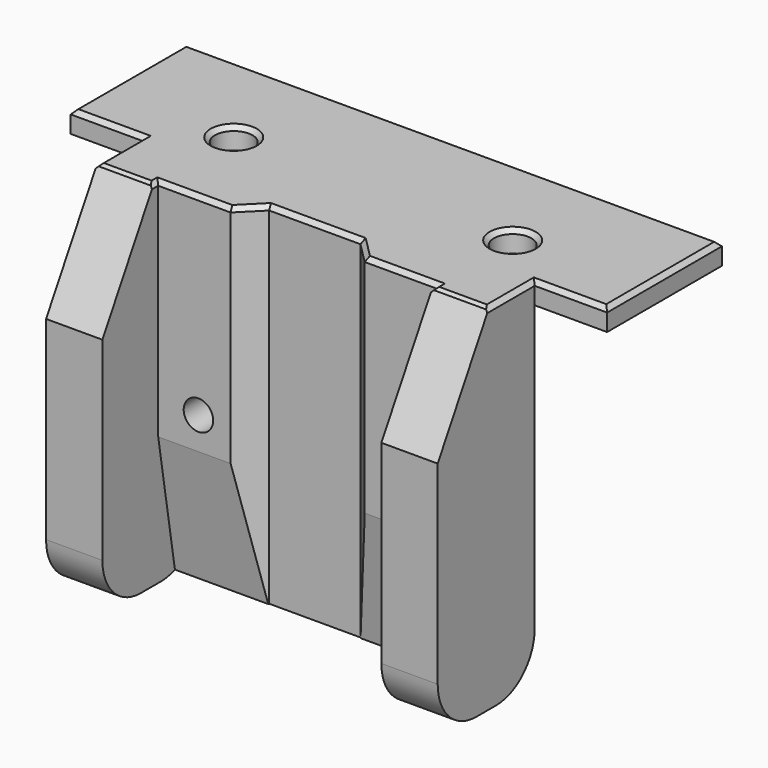
from build123d import *

# Parameters (mm, degrees)
F0_W           = 13.375
F0_H           = 2
F1_DEPTH       = 25
F2_R           = 1.75
F3_DEPTH       = 2
F4_W           = 11.3
F4_H           = 33
F5_DEPTH       = 18.25
F6_W           = 26
F6_H           = 6.5
F7_DEPTH       = 33
F9_DEPTH       = 33
F11_DEPTH      = 13
F11_DEPTH_BACK = 13
F12_R          = 1.375
F13_DEPTH      = 4.8
F14_W          = 5.5
F14_H          = 5.5
F15_DEPTH      = 1.5
F16_T1_DEPTH   = 27.75
F16_T3_DEPTH   = 27.75
F16_T5_DEPTH   = 59
F17_T1_DEPTH   = 59.021567647
F17_T3_DEPTH   = 59.021567647
F18_T1_DEPTH   = 15.4323463904
F18_T3_DEPTH   = 52.0573463904
F18_T5_DEPTH   = 7.7786731952
F18_T7_DEPTH   = 6.3286731952
F18_T9_DEPTH   = 6.4746360003
F18_T11_DEPTH  = 1.5286731952
F18_T13_DEPTH  = 7.7786731952
F18_T15_DEPTH  = 7.7786731952
F18_T17_DEPTH  = 6.4746360003
F18_T19_DEPTH  = 7.7786731952
F18_T24_DEPTH  = 4.8857735151
F18_T29_DEPTH  = 10.5573463904
F18_T35_DEPTH  = 4.8857735151
F18_T45_DEPTH  = 7.7786731952
F18_T49_DEPTH  = 7.3573463904
F18_T56_DEPTH  = 2.5573463904
F18_T60_DEPTH  = 8.8073463904
F18_T67_DEPTH  = 10.5573463904
F18_T71_DEPTH  = 4.8857735151
F18_T78_DEPTH  = 4.8857735151
F18_T82_DEPTH  = 10.5573463904
F18_T89_DEPTH  = 2.5573463904
F18_T93_DEPTH  = 8.8073463904
F18_T100_DEPTH = 7.7786731952
F18_T104_DEPTH = 7.3573463904


# Not quite as in the source:
# - a fillet or chamfer that OpenCascade refuses, or shapes differently, is made with other operations: its cross-section is extruded or revolved along the edge and cut away or added


with BuildPart() as f1:
    # F0 (on Right) → F1 (new body, symmetric)
    with BuildSketch(Plane.YZ):
        with Locations((6.6875, 1)):
            Rectangle(F0_W, F0_H)
    extrude(amount=F1_DEPTH, both=True)

    # F2 (on face) → F3 (cut, through all)
    with BuildSketch(Plane.XY.offset(2)):
        with Locations((-13, 4)):
            Circle(F2_R)
        with Locations((13, 4)):
            Circle(F2_R)
    extrude(amount=-F3_DEPTH, mode=Mode.SUBTRACT)

    # F4 (on Right) → F5 (join, symmetric)
    with BuildSketch(Plane.YZ):
        with Locations((-5.65, -14.5)):
            Rectangle(F4_W, F4_H)
    extrude(amount=F5_DEPTH, both=True)

    # F6 (on face) → F7 (cut, through all)
    with BuildSketch(Plane(origin=(0, 0, -31), x_dir=(1, 0, 0), z_dir=(0, 0, -1))):
        with Locations((0, 8.05)):
            Rectangle(F6_W, F6_H)
    extrude(amount=-F7_DEPTH, mode=Mode.SUBTRACT)

    # F8 (on face) → F9 (cut, through all)
    with BuildSketch(Plane(origin=(0, 0, -31), x_dir=(1, 0, 0), z_dir=(0, 0, -1))):
        Polygon((6.25, 4.8), (-6.25, 4.8), (-4.25, 2.8), (4.25, 2.8), align=None)
    extrude(amount=-F9_DEPTH, mode=Mode.SUBTRACT)

    # F10 (on Right) → F11 (cut, two sides)
    with BuildSketch(Plane.YZ) as f11_sk:
        Polygon((-4.8, -31), (-2.8, -31), (-4.8, -19), align=None)
    extrude(amount=F11_DEPTH, mode=Mode.SUBTRACT)
    extrude(f11_sk.sketch, amount=-F11_DEPTH_BACK, mode=Mode.SUBTRACT)

    # F12 (on face) → F13 (cut, through all)
    with BuildSketch(Plane.XZ.offset(4.8)):
        with Locations((-9.25, -16)):
            Circle(F12_R)
        with Locations((9.25, -16)):
            Circle(F12_R)
    extrude(amount=-F13_DEPTH, mode=Mode.SUBTRACT)

    # F14 (on face) → F15 (cut)
    with BuildSketch(Plane(origin=(0, 0, 0), x_dir=(-1, 0, 0), z_dir=(0, 1, 0))):
        with Locations((-9.25, -16)):
            Rectangle(F14_W, F14_H)
        with Locations((9.25, -16)):
            Rectangle(F14_W, F14_H)
    extrude(amount=-F15_DEPTH, mode=Mode.SUBTRACT)

    # F16: fillet of radius 4.5 on 3 edges, made by hand

    # F16_s2 → F16_t1 (cut)
    with BuildSketch(Plane.YZ.offset(-29.5)):
        with BuildLine():
            ThreePointArc((-11.3, -26.5), (-9.9819805153, -29.6819805153), (-6.8, -31))
            Line((-6.8, -31), (-11.3, -31))
            Line((-11.3, -31), (-11.3, -26.5))
        make_face()
    extrude(amount=F16_T1_DEPTH, mode=Mode.SUBTRACT)

    # F16_s4 → F16_t3 (cut)
    with BuildSketch(Plane.YZ.offset(1.75)):
        with BuildLine():
            ThreePointArc((-11.3, -26.5), (-9.9819805153, -29.6819805153), (-6.8, -31))
            Line((-6.8, -31), (-11.3, -31))
            Line((-11.3, -31), (-11.3, -26.5))
        make_face()
    extrude(amount=F16_T3_DEPTH, mode=Mode.SUBTRACT)

    # F16_s6 → F16_t5 (cut)
    with BuildSketch(Plane.YZ.offset(-29.5)):
        with BuildLine():
            ThreePointArc((0, -26.5), (-1.3180194847, -29.6819805153), (-4.5, -31))
            Line((-4.5, -31), (0, -31))
            Line((0, -31), (0, -26.5))
        make_face()
    extrude(amount=F16_T5_DEPTH, mode=Mode.SUBTRACT)

    # F17: chamfer of 6 x 10.3923048454 on 2 edges, made by hand

    # F17_s2 → F17_t1 (cut)
    with BuildSketch(Plane.YZ.offset(-45.1357838235)):
        Polygon((-5.3, 2), (-11.3, -8.3923048454), (-11.3, 2), align=None)
    extrude(amount=F17_T1_DEPTH, mode=Mode.SUBTRACT)

    # F17_s4 → F17_t3 (cut)
    with BuildSketch(Plane.YZ.offset(-13.8857838235)):
        Polygon((-5.3, 2), (-11.3, -8.3923048454), (-11.3, 2), align=None)
    extrude(amount=F17_T3_DEPTH, mode=Mode.SUBTRACT)

    # F18: chamfer of 0.4 on 18 edges, made by hand

    # F18_s2 → F18_t1 (cut)
    with BuildSketch(Plane.XZ.offset(-14.4036731952)):
        Polygon((25, 1.6), (24.6, 2), (25, 2), align=None)
        Polygon((-25, 1.6), (-24.6, 2), (-25, 2), align=None)
    extrude(amount=F18_T1_DEPTH, mode=Mode.SUBTRACT)

    # F18_s4 → F18_t3 (cut)
    with BuildSketch(Plane.YZ.offset(-26.0286731952)):
        Polygon((13.375, 1.6), (12.975, 2), (13.375, 2), align=None)
    extrude(amount=F18_T3_DEPTH, mode=Mode.SUBTRACT)

    # F18_s6 → F18_t5 (cut)
    with BuildSketch(Plane.YZ.offset(-26.0286731952)):
        Polygon((0, 1.6), (0.4, 2), (0, 2), align=None)
    extrude(amount=F18_T5_DEPTH, mode=Mode.SUBTRACT)

    # F18_s8 → F18_t7 (cut)
    with BuildSketch(Plane.XZ):
        Polygon((-18.25, 1.6), (-17.85, 2), (-18.25, 2), align=None)
        Polygon((18.25, 1.6), (17.85, 2), (18.25, 2), align=None)
    extrude(amount=F18_T7_DEPTH, mode=Mode.SUBTRACT)

    # F18_s10 → F18_t9 (cut)
    with BuildSketch(Plane.YZ.offset(-18.8623180002)):
        Polygon((-5.4154700538, 1.8), (-5.0690598923, 2), (-5.3, 2), align=None)
    extrude(amount=F18_T9_DEPTH, mode=Mode.SUBTRACT)

    # F18_s12 → F18_t11 (cut)
    with BuildSketch(Plane.XZ.offset(4.8)):
        Polygon((-13, 1.6), (-13.4, 2), (-13, 2), align=None)
        Polygon((13, 1.6), (13.4, 2), (13, 2), align=None)
    extrude(amount=F18_T11_DEPTH, mode=Mode.SUBTRACT)

    # F18_s14 → F18_t13 (cut)
    with BuildSketch(Plane.YZ.offset(-13)):
        Polygon((-4.8, 1.6), (-4.4, 2), (-4.8, 2), align=None)
    extrude(amount=F18_T13_DEPTH, mode=Mode.SUBTRACT)

    # F18_s16 → F18_t15 (cut)
    with BuildSketch(Plane.YZ.offset(5.2213268048)):
        Polygon((-4.8, 1.6), (-4.4, 2), (-4.8, 2), align=None)
    extrude(amount=F18_T15_DEPTH, mode=Mode.SUBTRACT)

    # F18_s18 → F18_t17 (cut)
    with BuildSketch(Plane.YZ.offset(12.3876819998)):
        Polygon((-5.4154700538, 1.8), (-5.0690598923, 2), (-5.3, 2), align=None)
    extrude(amount=F18_T17_DEPTH, mode=Mode.SUBTRACT)

    # F18_s20 → F18_t19 (cut)
    with BuildSketch(Plane.YZ.offset(18.25)):
        Polygon((0, 1.6), (0.4, 2), (0, 2), align=None)
    extrude(amount=F18_T19_DEPTH, mode=Mode.SUBTRACT)


with BuildPart() as f18_tool22:
    # F18_s23 → F18_t24 (new body)
    with BuildSketch(Plane(origin=(-6.2523817919, -6.2523817919, 0), x_dir=(0, 0, 1), z_dir=(0.7071067812, 0.7071067812, 0))):
        Polygon((1.6, -1.0253048327), (2, -1.4253048327), (2, -1.0253048327), align=None)
    extrude(amount=F18_T24_DEPTH)

    split(bisect_by=Plane.XZ.offset(2.8), keep=Keep.TOP)


with BuildPart() as f1_1:
    add(f1.part)

    # F18_t21: cut F18_tool22
    add(f18_tool22.part, mode=Mode.SUBTRACT)


with BuildPart() as f18_tool27:
    # F18_s28 → F18_t29 (new body)
    with BuildSketch(Plane.YZ.offset(-5.2786731952)):
        Polygon((-2.8, 1.6), (-2.4, 2), (-2.8, 2), align=None)
    extrude(amount=F18_T29_DEPTH)

    split(bisect_by=Plane(origin=(0.725, 0.725, 0), x_dir=(0, 0, 1), z_dir=(-0.7071067812, -0.7071067812, 0)), keep=Keep.TOP)

    split(bisect_by=Plane(origin=(-0.725, 0.725, 0), x_dir=(0, 0, 1), z_dir=(0.7071067812, -0.7071067812, 0)), keep=Keep.TOP)


with BuildPart() as f1_2:
    add(f1_1.part)

    # F18_t26: cut F18_tool27
    add(f18_tool27.part, mode=Mode.SUBTRACT)


with BuildPart() as f18_tool33:
    # F18_s34 → F18_t35 (new body)
    with BuildSketch(Plane(origin=(2.7976182081, -2.7976182081, 0), x_dir=(0, 0, 1), z_dir=(0.7071067812, -0.7071067812, 0))):
        Polygon((1.6, -1.0253048327), (2, -1.4253048327), (2, -1.0253048327), align=None)
    extrude(amount=F18_T35_DEPTH)

    split(bisect_by=Plane.XZ.offset(2.8), keep=Keep.TOP)


with BuildPart() as f1_3:
    add(f1_2.part)

    # F18_t32: cut F18_tool33
    add(f18_tool33.part, mode=Mode.SUBTRACT)

    # F18_s37 → F18_t38 (revolve, cut)
    with BuildSketch(Plane.XZ.offset(-4)):
        Polygon((-11.25, 1.6), (-10.85, 2), (-11.25, 2), align=None)
    revolve(axis=Axis((-13, 4, 2), (0, 0, 1)), mode=Mode.SUBTRACT)

    # F18_s39 → F18_t40 (revolve, cut)
    with BuildSketch(Plane.XZ.offset(-4)):
        Polygon((14.75, 1.6), (15.15, 2), (14.75, 2), align=None)
    revolve(axis=Axis((13, 4, 2), (0, 0, 1)), mode=Mode.SUBTRACT)


with BuildPart() as f18_tool43:
    # F18_s44 → F18_t45 (new body)
    with BuildSketch(Plane.YZ.offset(-17.2213268048)):
        Polygon((0, 1.6), (0.4, 2), (0, 2), align=None)
    extrude(amount=-F18_T45_DEPTH)

    split(bisect_by=Plane.YZ.offset(-18.25), keep=Keep.TOP)


with BuildPart() as f18_tool47:
    # F18_s48 → F18_t49 (new body)
    with BuildSketch(Plane.XZ.offset(-1.0286731952)):
        Polygon((-18.25, 1.6), (-17.85, 2), (-18.25, 2), align=None)
    extrude(amount=F18_T49_DEPTH)

    split(bisect_by=Plane.XZ, keep=Keep.BOTTOM)


with BuildPart() as f18_tool43_1:
    add(f18_tool43.part)

    # F18_t51: intersect F18_tool47
    add(f18_tool47.part, mode=Mode.INTERSECT)


with BuildPart() as f1_4:
    add(f1_3.part)

    # F18_t41: cut F18_tool43
    add(f18_tool43_1.part, mode=Mode.SUBTRACT)


with BuildPart() as f18_tool54:
    # F18_s55 → F18_t56 (new body)
    with BuildSketch(Plane.XZ.offset(6.3286731952)):
        Polygon((-13, 1.6), (-13.4, 2), (-13, 2), align=None)
    extrude(amount=-F18_T56_DEPTH)

    split(bisect_by=Plane.XZ.offset(4.8), keep=Keep.BOTTOM)


with BuildPart() as f18_tool58:
    # F18_s59 → F18_t60 (new body)
    with BuildSketch(Plane.YZ.offset(-14.0286731952)):
        Polygon((-4.8, 1.6), (-4.4, 2), (-4.8, 2), align=None)
    extrude(amount=F18_T60_DEPTH)

    split(bisect_by=Plane.YZ.offset(-13), keep=Keep.BOTTOM)


with BuildPart() as f18_tool54_1:
    add(f18_tool54.part)

    # F18_t62: intersect F18_tool58
    add(f18_tool58.part, mode=Mode.INTERSECT)


with BuildPart() as f1_5:
    add(f1_4.part)

    # F18_t52: cut F18_tool54
    add(f18_tool54_1.part, mode=Mode.SUBTRACT)


with BuildPart() as f18_tool65:
    # F18_s66 → F18_t67 (new body)
    with BuildSketch(Plane.YZ.offset(-5.2786731952)):
        Polygon((-2.8, 1.6), (-2.4, 2), (-2.8, 2), align=None)
    extrude(amount=F18_T67_DEPTH)

    split(bisect_by=Plane(origin=(-0.725, 0.725, 0), x_dir=(0, 0, 1), z_dir=(-0.7071067812, 0.7071067812, 0)), keep=Keep.TOP)


with BuildPart() as f18_tool69:
    # F18_s70 → F18_t71 (new body)
    with BuildSketch(Plane(origin=(-6.2523817919, -6.2523817919, 0), x_dir=(0, 0, 1), z_dir=(0.7071067812, 0.7071067812, 0))):
        Polygon((1.6, -1.0253048327), (2, -1.4253048327), (2, -1.0253048327), align=None)
    extrude(amount=F18_T71_DEPTH)

    split(bisect_by=Plane.XZ.offset(2.8), keep=Keep.BOTTOM)


with BuildPart() as f18_tool65_1:
    add(f18_tool65.part)

    # F18_t73: intersect F18_tool69
    add(f18_tool69.part, mode=Mode.INTERSECT)


with BuildPart() as f1_6:
    add(f1_5.part)

    # F18_t63: cut F18_tool65
    add(f18_tool65_1.part, mode=Mode.SUBTRACT)


with BuildPart() as f18_tool76:
    # F18_s77 → F18_t78 (new body)
    with BuildSketch(Plane(origin=(2.7976182081, -2.7976182081, 0), x_dir=(0, 0, 1), z_dir=(0.7071067812, -0.7071067812, 0))):
        Polygon((1.6, -1.0253048327), (2, -1.4253048327), (2, -1.0253048327), align=None)
    extrude(amount=F18_T78_DEPTH)

    split(bisect_by=Plane.XZ.offset(2.8), keep=Keep.BOTTOM)


with BuildPart() as f18_tool80:
    # F18_s81 → F18_t82 (new body)
    with BuildSketch(Plane.YZ.offset(-5.2786731952)):
        Polygon((-2.8, 1.6), (-2.4, 2), (-2.8, 2), align=None)
    extrude(amount=F18_T82_DEPTH)

    split(bisect_by=Plane(origin=(0.725, 0.725, 0), x_dir=(0, 0, 1), z_dir=(0.7071067812, 0.7071067812, 0)), keep=Keep.TOP)


with BuildPart() as f18_tool76_1:
    add(f18_tool76.part)

    # F18_t84: intersect F18_tool80
    add(f18_tool80.part, mode=Mode.INTERSECT)


with BuildPart() as f1_7:
    add(f1_6.part)

    # F18_t74: cut F18_tool76
    add(f18_tool76_1.part, mode=Mode.SUBTRACT)


with BuildPart() as f18_tool87:
    # F18_s88 → F18_t89 (new body)
    with BuildSketch(Plane.XZ.offset(3.7713268048)):
        Polygon((13, 1.6), (13.4, 2), (13, 2), align=None)
    extrude(amount=F18_T89_DEPTH)

    split(bisect_by=Plane.XZ.offset(4.8), keep=Keep.BOTTOM)


with BuildPart() as f18_tool91:
    # F18_s92 → F18_t93 (new body)
    with BuildSketch(Plane.YZ.offset(5.2213268048)):
        Polygon((-4.8, 1.6), (-4.4, 2), (-4.8, 2), align=None)
    extrude(amount=F18_T93_DEPTH)

    split(bisect_by=Plane.YZ.offset(13), keep=Keep.TOP)


with BuildPart() as f18_tool87_1:
    add(f18_tool87.part)

    # F18_t95: intersect F18_tool91
    add(f18_tool91.part, mode=Mode.INTERSECT)


with BuildPart() as f1_8:
    add(f1_7.part)

    # F18_t85: cut F18_tool87
    add(f18_tool87_1.part, mode=Mode.SUBTRACT)


with BuildPart() as f18_tool98:
    # F18_s99 → F18_t100 (new body)
    with BuildSketch(Plane.YZ.offset(25)):
        Polygon((0, 1.6), (0.4, 2), (0, 2), align=None)
    extrude(amount=-F18_T100_DEPTH)

    split(bisect_by=Plane.YZ.offset(18.25), keep=Keep.BOTTOM)


with BuildPart() as f18_tool102:
    # F18_s103 → F18_t104 (new body)
    with BuildSketch(Plane.XZ.offset(-1.0286731952)):
        Polygon((18.25, 1.6), (17.85, 2), (18.25, 2), align=None)
    extrude(amount=F18_T104_DEPTH)

    split(bisect_by=Plane.XZ, keep=Keep.BOTTOM)


with BuildPart() as f18_tool98_1:
    add(f18_tool98.part)

    # F18_t106: intersect F18_tool102
    add(f18_tool102.part, mode=Mode.INTERSECT)


with BuildPart() as f1_9:
    add(f1_8.part)

    # F18_t96: cut F18_tool98
    add(f18_tool98_1.part, mode=Mode.SUBTRACT)


solid = f1_9.part
